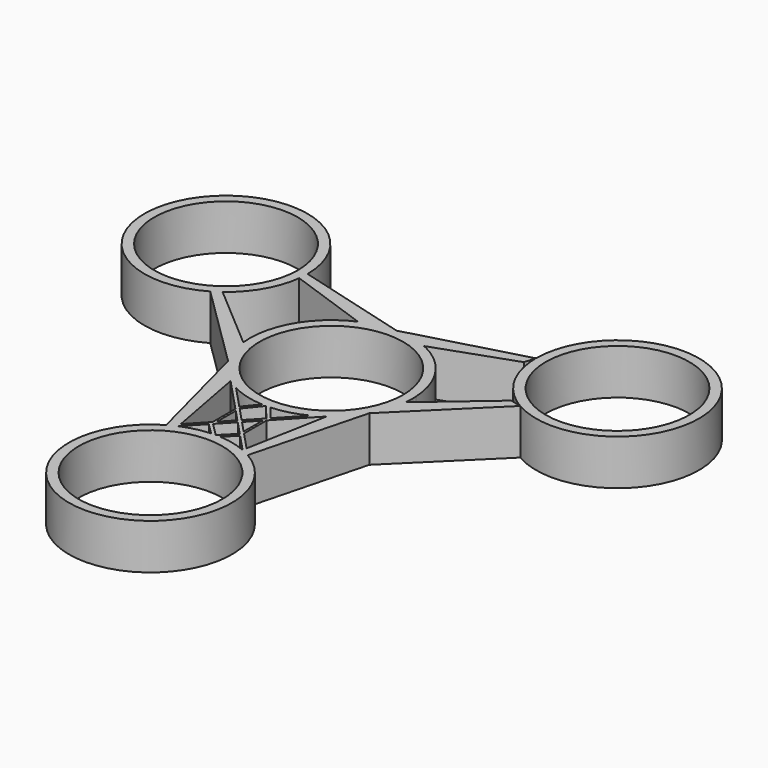
from build123d import *

# Parameters (mm, degrees)
F0_R     = 11.0625
F1_DEPTH = 7
F2_DEPTH = 7
F3_DEPTH = 7


# Not quite as in the source:
# - ends of sketch curves that miss each other by under 0.0002 mm in the source are joined


with BuildPart() as f1:
    # F0 (on Top) → F1 (new body)
    with BuildSketch(Plane.XY):
        with BuildLine():
            ThreePointArc((-22.6345681923, 7.3529683934), (-23.2441620991, 6.9245708082), (-23.878080543, 6.5330652161))
            Line((-23.878080543, 6.5330652161), (-10.879445222, -6.2812481173))
            ThreePointArc((-10.879445222, -6.2812481173), (-11.9437306049, -3.894060283), (-12.4910099647, -1.3383109926))
            Line((-12.4910099647, -1.3383109926), (-22.6345681923, 7.3529683934))
        make_face()
        with BuildLine():
            ThreePointArc((-17.6851304944, 15.925639103), (-17.6189235491, 16.6677649143), (-17.5968286604, 17.4125104381))
            ThreePointArc((-17.5968286604, 17.4125104381), (-41.0387722519, 23.6937613794), (-23.878080543, 6.5330652161))
            ThreePointArc((-23.878080543, 6.5330652161), (-23.2441620991, 6.9245708082), (-22.6345681923, 7.3529683934))
            ThreePointArc((-22.6345681923, 7.3529683934), (-19.2798866993, 11.1312566727), (-17.6851304944, 15.925639103))
        make_face()
        with Locations((-30.1593286604, 17.4125104381)):
            Circle(F0_R, mode=Mode.SUBTRACT)
        with BuildLine():
            Line((6.5218e-06, 12.5625), (-17.5968286604, 17.4125039163))
            ThreePointArc((-17.5968286604, 17.4125039163), (-17.6189235491, 16.6677649143), (-17.6851304944, 15.925639103))
            Line((-17.6851304944, 15.925639103), (-5.0864857136, 11.4866909655))
            ThreePointArc((-5.0864857136, 11.4866909655), (-2.5995016661, 12.2906060607), (6.5218e-06, 12.5625))
        make_face()
        with BuildLine():
            ThreePointArc((5.0864976401, 11.4866856842), (2.5995144273, 12.2906033616), (6.5218e-06, 12.5625))
            ThreePointArc((6.5218e-06, 12.5625), (-2.5995016661, 12.2906060607), (-5.0864857136, 11.4866909655))
            ThreePointArc((-5.0864857136, 11.4866909655), (-10.8794419611, 6.2812537653), (-12.4910099647, -1.3383109926))
            ThreePointArc((-12.4910099647, -1.3383109926), (-11.9437306049, -3.894060283), (-10.879445222, -6.2812481173))
            ThreePointArc((-10.879445222, -6.2812481173), (-9.3442233374, -8.3965407443), (-7.4045198124, -10.1483738893))
            ThreePointArc((-7.4045198124, -10.1483738893), (-6.5874472871, -10.6968193632), (-5.729952579, -11.1796265453))
            ThreePointArc((-5.729952579, -11.1796265453), (-3.2590434265, -12.1323963912), (-0.6433064868, -12.546017815))
            ThreePointArc((-0.6433064868, -12.546017815), (-0.3217587988, -12.5583787777), (0, -12.5625))
            ThreePointArc((0, -12.5625), (0.3217590306, -12.5583787718), (0.64330695, -12.5460177912))
            ThreePointArc((0.64330695, -12.5460177912), (3.2590426993, -12.1323965866), (5.7299508261, -11.1796274437))
            ThreePointArc((5.7299508261, -11.1796274437), (6.5874457148, -10.6968203315), (7.4045184202, -10.1483749051))
            ThreePointArc((7.4045184202, -10.1483749051), (9.3442190031, -8.3965455678), (10.879439599, -6.2812578567))
            ThreePointArc((10.879439599, -6.2812578567), (11.9437270351, -3.894071232), (12.491008709, -1.3383227122))
            ThreePointArc((12.491008709, -1.3383227122), (12.5446144452, -0.6701154167), (12.5625, 0))
            ThreePointArc((12.5625, 0), (12.5585786957, 0.3138588742), (12.546817231, 0.6275218102))
            ThreePointArc((12.546817231, 0.6275218102), (10.8794485026, 6.2812424352), (6.816873119, 10.5520920736))
            ThreePointArc((6.816873119, 10.5520920736), (5.9700021073, 11.0533018184), (5.0864976401, 11.4866856842))
        make_face()
        Circle(F0_R, mode=Mode.SUBTRACT)
        with BuildLine():
            Line((17.5968467396, 17.4124856456), (6.5218e-06, 12.5625))
            ThreePointArc((6.5218e-06, 12.5625), (2.5995144273, 12.2906033616), (5.0864976401, 11.4866856842))
            Line((5.0864976401, 11.4866856842), (17.0859847543, 15.7145153795))
            Line((17.0859847543, 15.7145153795), (17.5968467396, 17.4124856456))
        make_face()
        with BuildLine():
            Line((10.879439599, -6.2812578567), (23.8780929743, 6.5330371628))
            Line((23.8780929743, 6.5330371628), (22.1521745654, 6.9396060316))
            Line((22.1521745654, 6.9396060316), (12.491008709, -1.3383227122))
            ThreePointArc((12.491008709, -1.3383227122), (11.9437270351, -3.894071232), (10.879439599, -6.2812578567))
        make_face()
        with BuildLine():
            ThreePointArc((-4.9494347308, -23.2785935419), (-5.6252349846, -23.5923183247), (-6.2812481173, -23.945554778))
            ThreePointArc((-6.2812481173, -23.945554778), (-6.2812509413, -45.7044435916), (12.5625, -34.825))
            ThreePointArc((12.5625, -34.825), (10.879445222, -28.5437518827), (6.2812537653, -23.9455580389))
            ThreePointArc((6.2812537653, -23.9455580389), (5.6252404686, -23.5923210711), (4.949440011, -23.2785958053))
            ThreePointArc((4.949440011, -23.2785958053), (2.8710438959, -22.5949749306), (0.7055599905, -22.282329178))
            ThreePointArc((0.7055599905, -22.282329178), (0.3529192884, -22.267458273), (0, -22.2625))
            ThreePointArc((0, -22.2625), (-0.3529192884, -22.267458273), (-0.7055599905, -22.282329178))
            ThreePointArc((-0.7055599905, -22.282329178), (-2.8710410995, -22.5949742742), (-4.9494347308, -23.2785935419))
        make_face()
        with Locations((0, -34.825)):
            Circle(F0_R, mode=Mode.SUBTRACT)
        with BuildLine():
            Line((6.2812537653, -23.9455580389), (10.879439599, -6.2812578567))
            ThreePointArc((10.879439599, -6.2812578567), (9.3442190031, -8.3965455678), (7.4045184202, -10.1483749051))
            Line((7.4045184202, -10.1483749051), (5.0661976857, -22.6541538095))
            Line((5.0661976857, -22.6541538095), (6.2812537653, -23.9455580389))
        make_face()
        with BuildLine():
            ThreePointArc((-7.4045198124, -10.1483738893), (-9.3442233374, -8.3965407443), (-10.879445222, -6.2812481173))
            Line((-10.879445222, -6.2812481173), (-6.2812481173, -23.945554778))
            Line((-6.2812481173, -23.945554778), (-5.0661928327, -22.6541510186))
            Line((-5.0661928327, -22.6541510186), (-7.4045198124, -10.1483738893))
        make_face()
        with BuildLine():
            ThreePointArc((4.949440011, -23.2785958053), (5.6252404686, -23.5923210711), (6.2812537653, -23.9455580389))
            Line((6.2812537653, -23.9455580389), (5.0661976857, -22.6541538095))
            Line((5.0661976857, -22.6541538095), (4.949440011, -23.2785958053))
        make_face()
        with BuildLine():
            Line((-5.0661928327, -22.6541510186), (-6.2812481173, -23.945554778))
            ThreePointArc((-6.2812481173, -23.945554778), (-5.6252349846, -23.5923183247), (-4.9494347308, -23.2785935419))
            Line((-4.9494347308, -23.2785935419), (-5.0661928327, -22.6541510186))
        make_face()
    extrude(amount=F1_DEPTH)

    # F0 (on Top) → F2 (join)
    with BuildSketch(Plane.XY):
        with BuildLine():
            Line((2.0575288422, -20.2049711578), (0, -22.2625))
            ThreePointArc((0, -22.2625), (0.3529192884, -22.267458273), (0.7055599905, -22.282329178))
            Line((0.7055599905, -22.282329178), (2.4091755513, -20.5787136171))
            Line((2.4091755513, -20.5787136171), (2.0575288422, -20.2049711578))
        make_face()
        with BuildLine():
            Line((-2.4091743081, -20.5787148604), (-0.7055599905, -22.282329178))
            ThreePointArc((-0.7055599905, -22.282329178), (-0.3529192884, -22.267458273), (0, -22.2625))
            Line((0, -22.2625), (-2.0575276516, -20.2049723484))
            Line((-2.0575276516, -20.2049723484), (-2.4091743081, -20.5787148604))
        make_face()
        Polygon((-2.0575276516, -19.4564351822), (-2.4091743081, -19.8301776941), (-2.4091743081, -20.5787148604), (-2.0575276516, -20.2049723484), align=None)
        Polygon((2.0575288422, -19.456435009), (2.0575288422, -20.2049711578), (2.4091755513, -20.5787136171), (2.4091755513, -19.8301774684), align=None)
        Polygon((2.0575288422, -15.8313446679), (2.4091755513, -15.4576021), (2.4091755513, -14.7090649338), (2.0575288422, -15.0828075016), align=None)
        Polygon((-2.4091743081, -14.709066195), (-2.4091743081, -15.4576023437), (-2.0575276516, -15.8313447471), (-2.0575276516, -15.0828085984), align=None)
        Polygon((-2.0575276516, -15.8313447471), (-2.4091743081, -15.4576023437), (-2.4091743081, -19.8301776941), (-2.0575276516, -19.4564351822), align=None)
        Polygon((2.4091755513, -19.8301774684), (2.4091755513, -15.4576021), (2.0575288422, -15.8313446679), (2.0575288422, -19.456435009), align=None)
        with BuildLine():
            ThreePointArc((0, -12.5625), (-0.3217587988, -12.5583787777), (-0.6433064868, -12.546017815))
            Line((-0.6433064868, -12.546017815), (-2.4091743081, -14.709066195))
            Line((-2.4091743081, -14.709066195), (-2.0575276516, -15.0828085984))
            Line((-2.0575276516, -15.0828085984), (0, -12.5625))
        make_face()
        with BuildLine():
            ThreePointArc((0.64330695, -12.5460177912), (0.3217590306, -12.5583787718), (0, -12.5625))
            Line((0, -12.5625), (2.0575288422, -15.0828075016))
            Line((2.0575288422, -15.0828075016), (2.4091755513, -14.7090649338))
            Line((2.4091755513, -14.7090649338), (0.64330695, -12.5460177912))
        make_face()
        Polygon((2.4091755513, -20.5787136171), (4.949440011, -23.2785958053), (5.0661976857, -22.6541538095), (2.4091755513, -19.8301774684), align=None)
        Polygon((-2.4091743081, -19.8301776941), (-5.0661928327, -22.6541510186), (-4.9494347308, -23.2785935419), (-2.4091743081, -20.5787148604), align=None)
        with BuildLine():
            Line((2.4091755513, -15.4576021), (7.4045184202, -10.1483749051))
            ThreePointArc((7.4045184202, -10.1483749051), (6.5874457148, -10.6968203315), (5.7299508261, -11.1796274437))
            Line((5.7299508261, -11.1796274437), (2.4091755513, -14.7090649338))
            Line((2.4091755513, -14.7090649338), (2.4091755513, -15.4576021))
        make_face()
        with BuildLine():
            ThreePointArc((-5.729952579, -11.1796265453), (-6.5874472871, -10.6968193632), (-7.4045198124, -10.1483738893))
            Line((-7.4045198124, -10.1483738893), (-2.4091743081, -15.4576023437))
            Line((-2.4091743081, -15.4576023437), (-2.4091743081, -14.709066195))
            Line((-2.4091743081, -14.709066195), (-5.729952579, -11.1796265453))
        make_face()
        Polygon((0.3521420553, -17.6438901016), (8.567e-07, -18.0181582303), (2.0575288422, -20.2049711578), (2.0575288422, -19.456435009), align=None)
        Polygon((3.781e-07, -17.2696215728), (-0.3521408205, -17.6438897015), (8.567e-07, -18.0181582303), (0.3521420553, -17.6438901016), align=None)
        Polygon((2.0575288422, -15.8313446679), (2.0575288422, -15.0828075016), (3.781e-07, -17.2696215728), (0.3521420553, -17.6438901016), align=None)
    extrude(amount=F2_DEPTH)

    # F0 (on Top) → F3 (join)
    with BuildSketch(Plane.XY):
        Polygon((-0.3521408205, -17.6438897015), (-2.0575276516, -19.4564351822), (-2.0575276516, -20.2049723484), (8.567e-07, -18.0181582303), align=None)
        Polygon((-2.0575276516, -15.0828085984), (-2.0575276516, -15.8313447471), (-0.3521408205, -17.6438897015), (3.781e-07, -17.2696215728), align=None)
    extrude(amount=F3_DEPTH)


with BuildPart() as f1b:
    # F0 (on Top) → F1, piece 2 (new body)
    with BuildSketch(Plane.XY):
        with BuildLine():
            ThreePointArc((42.7218467396, 17.4124791239), (30.1593500005, 29.9749791239), (17.5968467396, 17.4124856456))
            ThreePointArc((17.5968467396, 17.4124856456), (17.6189410484, 16.6677433655), (17.6851470299, 15.9256207407))
            ThreePointArc((17.6851470299, 15.9256207407), (18.1323107106, 13.7838691135), (18.9442912632, 11.7521843515))
            ThreePointArc((18.9442912632, 11.7521843515), (19.1077328162, 11.4393529795), (19.2798982567, 11.1312366546))
            ThreePointArc((19.2798982567, 11.1312366546), (19.4606516814, 10.8280785967), (19.6498504077, 10.5301181118))
            ThreePointArc((19.6498504077, 10.5301181118), (21.0033498024, 8.8110765443), (22.6345791818, 7.3529423825))
            ThreePointArc((22.6345791818, 7.3529423825), (23.2441737601, 6.9245437258), (23.8780929743, 6.5330371628))
            ThreePointArc((23.8780929743, 6.5330371628), (36.4405948569, 6.5330339019), (42.7218467396, 17.4124791239))
        make_face()
        with BuildLine():
            ThreePointArc((41.2218467396, 17.4124791239), (30.1593438681, 6.3499791239), (19.0968467396, 17.4124848669))
            ThreePointArc((19.0968467396, 17.4124848669), (30.1593496111, 28.4749791239), (41.2218467396, 17.4124791239))
        make_face(mode=Mode.SUBTRACT)
    extrude(amount=F1_DEPTH)


solid = Compound([f1.part, f1b.part])
